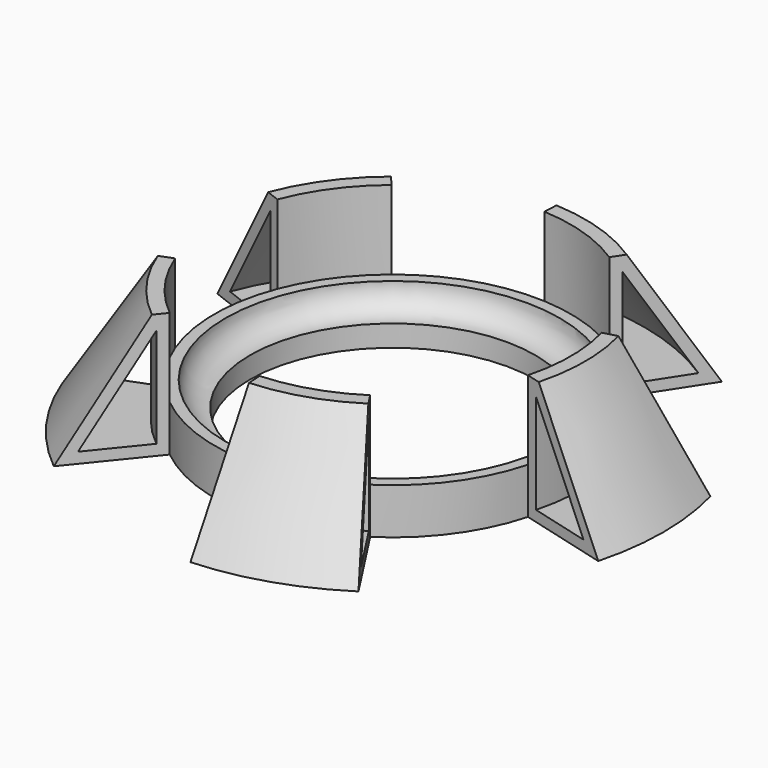
from build123d import *

# Parameters (mm, degrees)
F4_ANGLE_BACK   = 15
F4_ANGLE        = 30
F4_COPIES_COUNT = 5


# Not quite as in the source:
# - a pattern or mirror of a feature is missing from the dataset's text; its kind, count and spacing are read off the source's solid


with BuildPart() as f2:
    # F1 (on Front) → F2 (revolve)
    with BuildSketch(Plane.XZ):
        with BuildLine():
            Line((40, 6), (40, 0))
            Line((40, 0), (50, 0))
            Line((50, 0), (50, 12.9))
            Line((50, 12.9), (46.9, 12.9))
            ThreePointArc((46.9, 12.9), (44.8790367902, 8.0209632098), (40, 6))
        make_face()
    revolve(axis=Axis((0, 0, 7.8032705933), (0, 0, 1)))

    # F3 (on Front) → F4 (revolve)
    with BuildSketch(Plane.XZ, mode=Mode.PRIVATE) as f4_sk:
        Polygon((50, 35), (50, 0), (76, 0), (54, 35), align=None)
        Polygon((53, 30.9536291067), (70.5708525814, 3), (53, 3), align=None, mode=Mode.SUBTRACT)
    f4 = revolve(f4_sk.sketch.rotate(Axis((0, 0, 7.8032705933), (0, 0, 1)), -F4_ANGLE_BACK), axis=Axis((0, 0, 7.8032705933), (0, 0, 1)), revolution_arc=F4_ANGLE)

    # F4_copies: F4 ×5 about axis
    f4_copies_axis = Axis((0, 0, 0), (0, 0, 1))
    for i in range(1, F4_COPIES_COUNT):
        add(f4.rotate(f4_copies_axis, i * 360 / F4_COPIES_COUNT))


solid = f2.part
